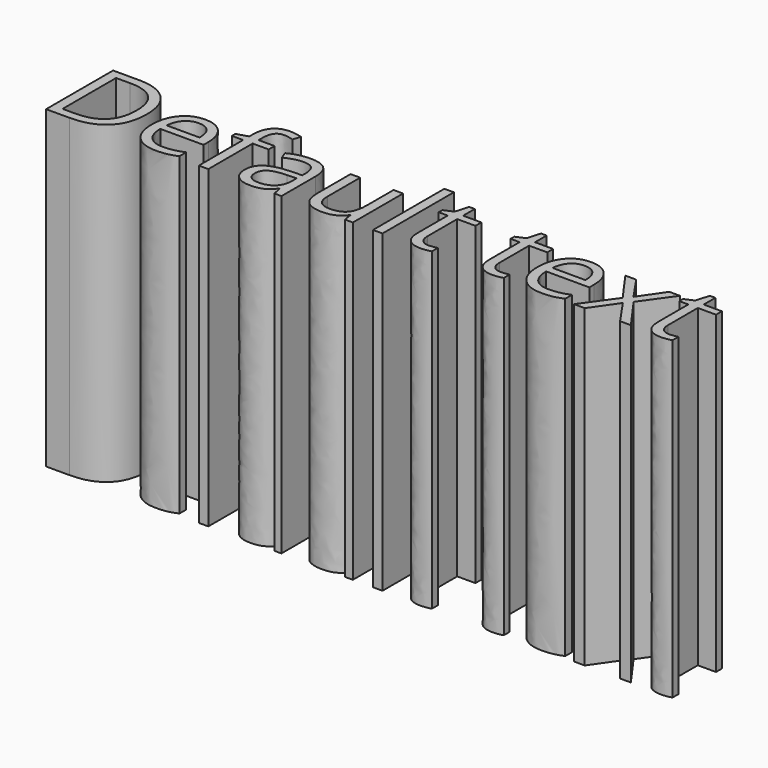
from build123d import *

# Parameters (mm, degrees)
F0_TEXT_SIZE = 9.4724456883
F1_DEPTH     = 25.4


# Not quite as in the source:
# - Text() gives the source's letters only with a copy of the font that has no kerning and outlines rounded to 1/6400 em; it was checked with that copy


with BuildPart() as f1:
    # F0 (on Top) → F1 (new body)
    with BuildSketch(Plane.XY):
        with Locations((0, -6.8201608956)):
            Text('Default text', F0_TEXT_SIZE, font='Open Sans', text_align=(TextAlign.LEFT, TextAlign.BOTTOM))
    extrude(amount=F1_DEPTH)


solid = f1.part
